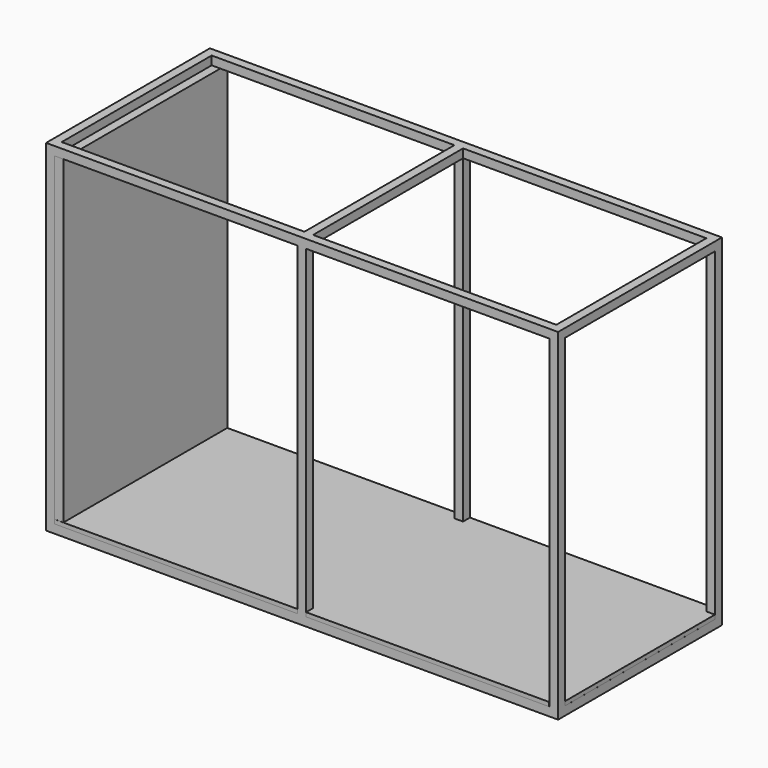
from build123d import *

# Parameters (mm, degrees)
F0_W      = 1500
F0_H      = 1000
F1_DEPTH  = 600
F2_W      = 711.9
F2_H      = 949.2
F2_W_2    = 25.4
F3_DEPTH  = 600.001
F4_W      = 549.2
F4_H      = 949.2
F5_DEPTH  = 1500.001
F6_W      = 1449.2
F6_H      = 549.2
F7_DEPTH  = 1000.001
F9_DEPTH  = 599.9734
F10_W     = 549.2
F10_H     = 949.2
F11_DEPTH = 1500.001
F13_DEPTH = 12
F14_W     = 600
F14_H     = 937.7431182263
F15_DEPTH = 25.4


with BuildPart() as f1:
    # F0 (on Front) → F1 (new body)
    with BuildSketch(Plane.XZ):
        with Locations((0.7634554058, -296.2822238567)):
            Rectangle(F0_W, F0_H)
    extrude(amount=F1_DEPTH)

    # F2 (on face) → F3 (cut, through all)
    with BuildSketch(Plane.XZ.offset(600)):
        with Locations((-367.8865445942, -296.2822238567)):
            Rectangle(F2_W, F2_H)
        with Locations((0.7634554058, -296.2822238567)):
            Rectangle(F2_W_2, F2_H)
        with Locations((369.4134554058, -296.2822238567)):
            Rectangle(F2_W, F2_H)
    extrude(amount=-F3_DEPTH, mode=Mode.SUBTRACT)

    # F4 (on face) → F5 (cut, through all)
    with BuildSketch(Plane(origin=(-749.2365445942, 0, 0), x_dir=(0, -1, 0), z_dir=(-1, 0, 0))):
        with Locations((300, -296.2822238567)):
            Rectangle(F4_W, F4_H)
    extrude(amount=-F5_DEPTH, mode=Mode.SUBTRACT)

    # F6 (on face) → F7 (cut, through all)
    with BuildSketch(Plane.XY.offset(203.7177761433)):
        with Locations((0.7634554058, -300)):
            Rectangle(F6_W, F6_H)
    extrude(amount=-F7_DEPTH, mode=Mode.SUBTRACT)

    # F8 (on face) → F9 (join)
    with BuildSketch(Plane.XZ.offset(600)):
        Polygon((12.7, 203.7177761433), (0, 203.7177761433), (-12.7, 203.7177761433), (-12.7, -796.2822238567), (12.7, -796.2822238567), align=None)
    extrude(amount=-F9_DEPTH)

    # F10 (on face) → F11 (cut, through all)
    with BuildSketch(Plane.YZ.offset(750.7634554058)):
        with Locations((-300, -296.2822238567)):
            Rectangle(F10_W, F10_H)
    extrude(amount=-F11_DEPTH, mode=Mode.SUBTRACT)


with BuildPart() as f13:
    # F12 (on face) → F13 (new body)
    with BuildSketch(Plane.XY.offset(-770.8822238567)):
        Polygon((-749.2365445942, -25.4), (-749.2365445942, -574.6), (-723.8365445942, -574.6), (-723.8365445942, -600.2621650696), (-12.8450281918, -600.2621650696), (-12.8450281918, -574.6), (12.7119384706, -574.6), (12.7119384706, -600.2621650696), (725.0914573669, -600.2621650696), (725.0914573669, -574.6), (750.7110238075, -574.6), (750.7110238075, -25.4), (725.0914573669, -25.4), (725.0914573669, 0), (12.7119384706, 0), (12.7119384706, -25.4), (-12.8450281918, -25.4), (-12.8450281918, 0), (-723.8365445942, 0), (-723.8365445942, -25.4), align=None)
    extrude(amount=F13_DEPTH)


with BuildPart() as f15:
    # F14 (on face) → F15 (new body)
    with BuildSketch(Plane.YZ.offset(-723.8365445942)):
        with Locations((-300, -290.5537829698)):
            Rectangle(F14_W, F14_H)
    extrude(amount=F15_DEPTH)


solid = Compound([f1.part, f13.part, f15.part])
